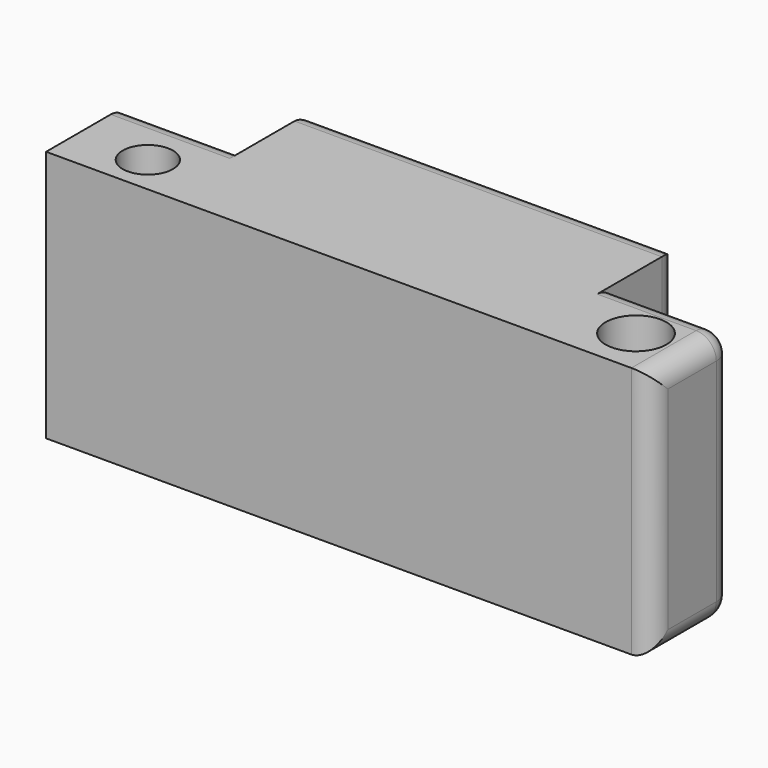
from build123d import *

# Parameters (mm, degrees)
F0_W         = 149.7976481915
F0_H         = 62.41568923
F1_DEPTH     = 25
F2_W         = 90.8637270331
F2_H         = 62.41568923
F3_DEPTH     = 20
F4_R         = 7.5225312021
F5_DEPTH     = 100
F6_R         = 6.2150283999
F7_DEPTH     = 100
F8_R         = 5
F9_T1_DEPTH  = 24.4669605792
F9_S5_W      = 5
F9_S5_H      = 5
F9_T6_DEPTH  = 5
F9_S11_W     = 5
F9_S11_H     = 5
F9_T12_DEPTH = 5
F10_R        = 5


# Not quite as in the source:
# - a fillet or chamfer that OpenCascade refuses, or shapes differently, is made with other operations: its cross-section is extruded or revolved along the edge and cut away or added


with BuildPart() as f1:
    # F0 (on Front) → F1 (new body)
    with BuildSketch(Plane.XZ):
        Rectangle(F0_W, F0_H)
    extrude(amount=F1_DEPTH)

    # F2 (on face) → F3 (join)
    with BuildSketch(Plane(origin=(0, 0, 0), x_dir=(-1, 0, 0), z_dir=(0, 1, 0))):
        Rectangle(F2_W, F2_H)
    extrude(amount=F3_DEPTH)

    # F4 (on face) → F5 (cut)
    with BuildSketch(Plane(origin=(0, 0, -31.207844615), x_dir=(1, 0, 0), z_dir=(0, 0, -1))):
        with Locations((61.5517050582, 13.1388221845)):
            Circle(F4_R)
    extrude(amount=-F5_DEPTH, mode=Mode.SUBTRACT)

    # F6 (on face) → F7 (cut)
    with BuildSketch(Plane.XY.offset(31.207844615)):
        with Locations((-57.4441173465, -15.3550794757)):
            Circle(F6_R)
    extrude(amount=-F7_DEPTH, mode=Mode.SUBTRACT)

    # F8
    f8_edges = [f1.edges().sort_by_distance(p)[0] for p in [
        (45.431864, 20, 0),
        (-45.431864, 20, 0),
        (74.898824, -12.5, -31.207845),
        (74.898824, -12.5, 31.207845),
        (74.898824, 0, 0),
        (74.898824, -25, 0),
        (0, 20, 31.207845),
        (0, 20, -31.207845),
    ]]
    fillet(f8_edges, radius=F8_R)

    # F9: fillet of radius 5 on 2 edges, made by hand

    # F9_s2 → F9_t1 (cut)
    with BuildSketch(Plane.YZ.offset(45.4318635166)):
        with BuildLine():
            ThreePointArc((-5, -31.207844615), (-1.4644660941, -29.7433785209), (0, -26.207844615))
            Line((0, -26.207844615), (0, -31.207844615))
            Line((0, -31.207844615), (-5, -31.207844615))
        make_face()
        with BuildLine():
            ThreePointArc((0, 26.207844615), (-1.4644660941, 29.7433785209), (-5, 31.207844615))
            Line((-5, 31.207844615), (0, 31.207844615))
            Line((0, 31.207844615), (0, 26.207844615))
        make_face()
    extrude(amount=F9_T1_DEPTH, mode=Mode.SUBTRACT)


with BuildPart() as f9_tool4:
    # F9_s5 → F9_t6 (new body)
    with BuildSketch(Plane.XZ.offset(5)):
        with Locations((72.3988240957, 28.707844615)):
            Rectangle(F9_S5_W, F9_S5_H)
    extrude(amount=-F9_T6_DEPTH)

    # F9_s7 → F9_t8 (revolve, cut)
    with BuildSketch(Plane(origin=(69.8988240957, -5, 26.207844615), x_dir=(-0.7071067812, 0, -0.7071067812), z_dir=(0.7071067812, 0, -0.7071067812))):
        with BuildLine():
            ThreePointArc((0, -5), (5, 0), (0, 5))
            Line((0, 5), (0, -5))
        make_face()
    revolve(axis=Axis((69.8988240957, -5, 26.207844615), (0, 1, 0)), mode=Mode.SUBTRACT)


with BuildPart() as f1_1:
    add(f1.part)

    # F9_t3: cut F9_tool4
    add(f9_tool4.part, mode=Mode.SUBTRACT)


with BuildPart() as f9_tool10:
    # F9_s11 → F9_t12 (new body)
    with BuildSketch(Plane.XY.offset(-26.207844615)):
        with Locations((72.3988240957, -2.5)):
            Rectangle(F9_S11_W, F9_S11_H)
    extrude(amount=-F9_T12_DEPTH)

    # F9_s13 → F9_t14 (revolve, cut)
    with BuildSketch(Plane(origin=(69.8988240957, -5, -26.207844615), x_dir=(-0.7071067812, -0.7071067812, 0), z_dir=(0.7071067812, -0.7071067812, 0))):
        with BuildLine():
            ThreePointArc((0, -5), (5, 0), (0, 5))
            Line((0, 5), (0, -5))
        make_face()
    revolve(axis=Axis((69.8988240957, -5, -26.207844615), (0, 0, -1)), mode=Mode.SUBTRACT)


with BuildPart() as f1_2:
    add(f1_1.part)

    # F9_t9: cut F9_tool10
    add(f9_tool10.part, mode=Mode.SUBTRACT)

    # F10
    f10_edges = [f1_2.edges().sort_by_distance(p)[0] for p in [
        (-60.165344, 0, -31.207845),
        (-60.165344, 0, 31.207845),
    ]]
    fillet(f10_edges, radius=F10_R)


solid = f1_2.part
